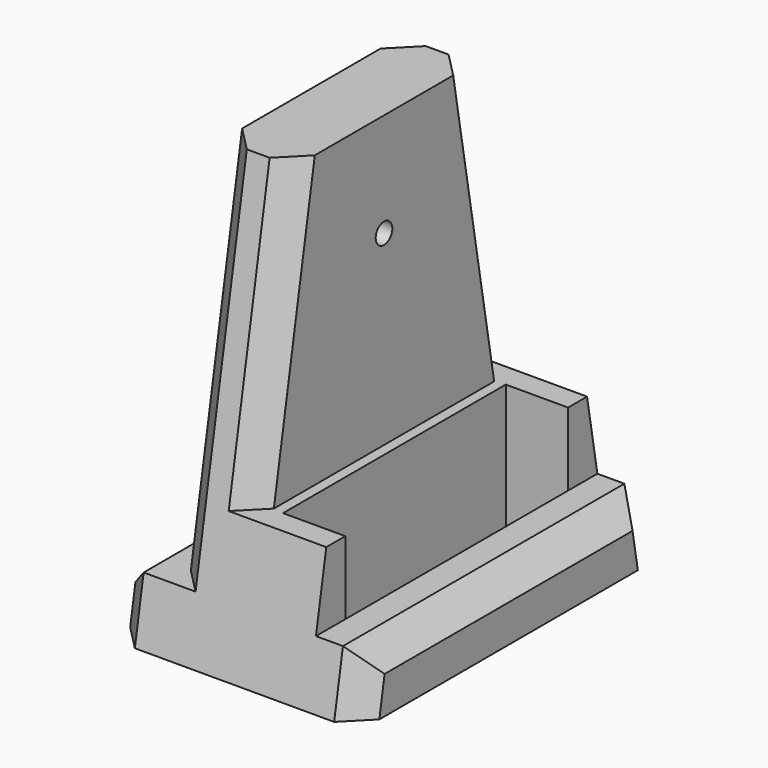
from build123d import *

# Parameters (mm, degrees)
F1_DEPTH = 90
F2_R     = 5
F3_DEPTH = 50
F4_W     = 30
F4_H     = 134.1311782598
F5_DEPTH = 40
F7_W     = 309.0550526977
F7_H     = 293.745405972
F8_DEPTH = 60
F9_SIZE  = 12


# Not quite as in the source:
# - a pattern or mirror of a feature is missing from the dataset's text; its kind, count and spacing are read off the source's solid


with BuildPart() as f1:
    # F0 (on Front) → F1 (new body, symmetric)
    with BuildSketch(Plane.XZ):
        Polygon((0, 65.2183964849), (0, 205), (-35, 205), (-35, 30), (-60, 30), (-60, 0), (0, 0), (60, 0), (60, 30), (35, 30), (35, 65.2183964849), align=None)
    extrude(amount=F1_DEPTH, both=True)

    # F2 (on Right) → F3 (cut, symmetric)
    with BuildSketch(Plane.YZ):
        with Locations((0, 155)):
            Circle(F2_R)
    extrude(amount=F3_DEPTH, both=True, mode=Mode.SUBTRACT)

    # F4 (on face) → F5 (cut, symmetric)
    with BuildSketch(Plane.XY.offset(30)):
        with Locations((20, 0)):
            Rectangle(F4_W, F4_H)
    extrude(amount=F5_DEPTH, both=True, mode=Mode.SUBTRACT)

    # F7 (on face) → F8 (cut)
    with BuildSketch(Plane(origin=(0, 87.2861679354, 15.3909064497), x_dir=(-1, 0, 0), z_dir=(0, 0.984807753, 0.1736481777))):
        with Locations((10.5363130569, 83.1948332489)):
            Rectangle(F7_W, F7_H)
    f8 = extrude(amount=F8_DEPTH, mode=Mode.SUBTRACT)

    # F8_copies: F8 across plane
    add(f8.mirror(Plane(origin=(0, 0, 0), x_dir=(0, 0, -1), z_dir=(0, -1, 0))), mode=Mode.SUBTRACT)

    # F9
    f9_edges = [f1.edges().sort_by_distance(p)[0] for p in [
        (0, 66.176603, 135.109198),
        (-35, 69.28158, 117.5),
        (-60, 87.355095, 15),
        (60, 87.355095, 15),
        (-60, 0, 30),
        (60, 0, 30),
        (0, -66.176603, 135.109198),
        (60, -87.355095, 15),
        (-35, -69.28158, 117.5),
        (-60, -87.355095, 15),
    ]]
    chamfer(f9_edges, length=F9_SIZE)


solid = f1.part
